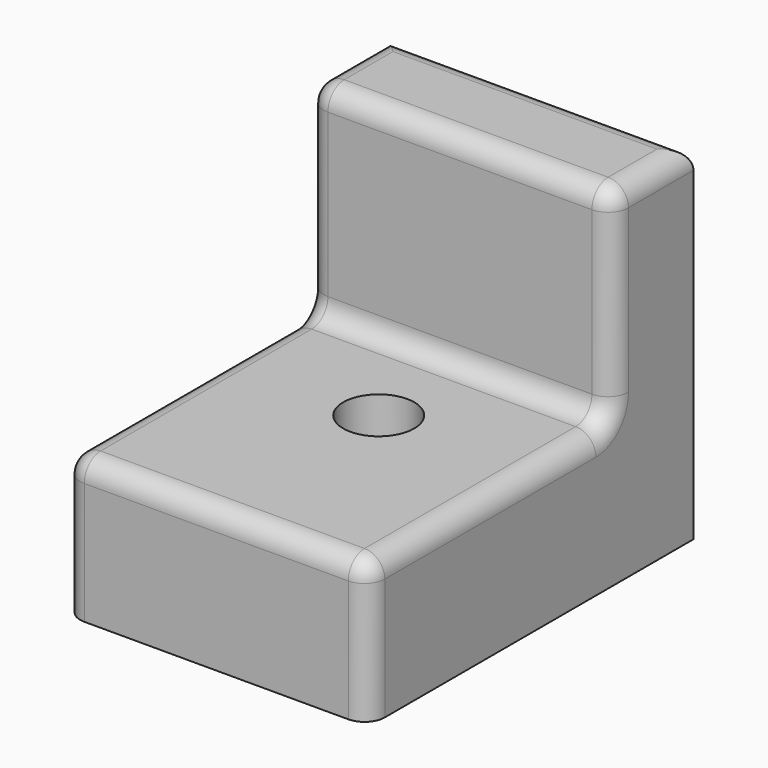
from build123d import *

# Parameters (mm, degrees)
F0_W     = 15
F0_H     = 20
F1_DEPTH = 17
F2_R     = 1.75
F3_DEPTH = 17.001
F2_W     = 15
F2_H     = 15
F4_DEPTH = 10
F5_R     = 1


with BuildPart() as f1:
    # F0 (on Top) → F1 (new body)
    with BuildSketch(Plane.XY):
        with Locations((-7.5, 10)):
            Rectangle(F0_W, F0_H)
    extrude(amount=F1_DEPTH)

    # F2 (on face) → F3 (cut, through all)
    with BuildSketch(Plane.XY.offset(17)):
        with Locations((-7.5, 10)):
            Circle(F2_R)
    extrude(amount=-F3_DEPTH, mode=Mode.SUBTRACT)

    # F2 (on face) → F4 (cut)
    with BuildSketch(Plane.XY.offset(17)):
        with Locations((-7.5, 7.5)):
            Rectangle(F2_W, F2_H)
        with Locations((-7.5, 10)):
            Circle(F2_R, mode=Mode.SUBTRACT)
    extrude(amount=-F4_DEPTH, mode=Mode.SUBTRACT)

    # F5
    f5_edges = [f1.edges().sort_by_distance(p)[0] for p in [
        (-7.5, 20, 17),
        (-7.5, 15, 17),
        (-7.5, 15, 7),
        (-7.5, 0, 7),
        (-15, 7.5, 7),
        (-15, 0, 3.5),
        (0, 15, 12),
        (0, 0, 3.5),
        (0, 17.5, 17),
        (-15, 17.5, 17),
        (0, 7.5, 7),
        (-15, 15, 12),
    ]]
    fillet(f5_edges, radius=F5_R)


solid = f1.part
